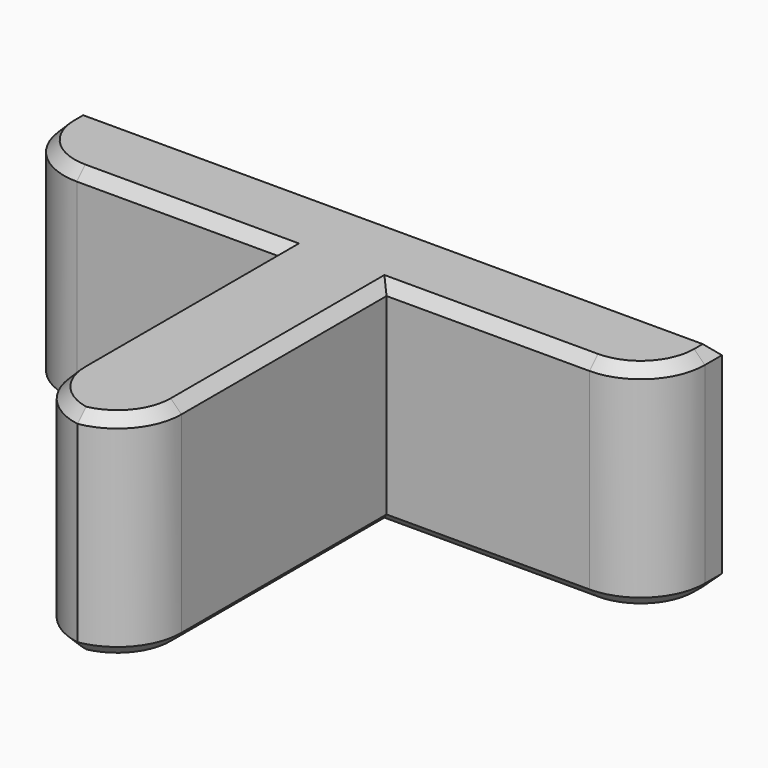
from build123d import *

# Parameters (mm, degrees)
F1_DEPTH    = 10
F2_T1_DEPTH = 25
F3_SIZE     = 0.5


# Not quite as in the source:
# - a fillet or chamfer that OpenCascade refuses, or shapes differently, is made with other operations: its cross-section is extruded or revolved along the edge and cut away or added


with BuildPart() as f1:
    # F0 (on Top) → F1 (new body)
    with BuildSketch(Plane.XY):
        Polygon((-15, 4), (-15, 0), (-2.5, 0), (-2.5, -15), (2.5, -15), (2.5, 0), (15, 0), (15, 4), align=None)
    extrude(amount=F1_DEPTH)

    # F2: fillet of radius 3 on 4 edges, made by hand

    # F2_s2 → F2_t1 (cut)
    with BuildSketch(Plane.XY.offset(-7.5)):
        with BuildLine():
            ThreePointArc((-2.5, -12), (-1.6213203436, -14.1213203436), (0.5, -15))
            Line((0.5, -15), (-2.5, -15))
            Line((-2.5, -15), (-2.5, -12))
        make_face()
        with BuildLine():
            ThreePointArc((-0.5, -15), (1.6213203436, -14.1213203436), (2.5, -12))
            Line((2.5, -12), (2.5, -15))
            Line((2.5, -15), (-0.5, -15))
        make_face()
        with BuildLine():
            ThreePointArc((-15, 3), (-14.1213203436, 0.8786796564), (-12, 0))
            Line((-12, 0), (-15, 0))
            Line((-15, 0), (-15, 3))
        make_face()
        with BuildLine():
            ThreePointArc((12, 0), (14.1213203436, 0.8786796564), (15, 3))
            Line((15, 3), (15, 0))
            Line((15, 0), (12, 0))
        make_face()
    extrude(amount=F2_T1_DEPTH, mode=Mode.SUBTRACT)

    # F3
    f3_edges = [f1.edges().sort_by_distance(p)[0] for p in [
        (0, 4, 10),
        (15, 3.5, 10),
        (14.12132, 0.87868, 10),
        (7.25, 0, 10),
        (2.5, -6, 10),
        (1.791288, -13.936492, 10),
        (-1.791288, -13.936492, 10),
        (-2.5, -6, 10),
        (-7.25, 0, 10),
        (-14.12132, 0.87868, 10),
        (-15, 3.5, 10),
        (0, 4, 0),
        (15, 3.5, 0),
        (14.12132, 0.87868, 0),
        (7.25, 0, 0),
        (2.5, -6, 0),
        (1.791288, -13.936492, 0),
        (-1.791288, -13.936492, 0),
        (-2.5, -6, 0),
        (-7.25, 0, 0),
        (-14.12132, 0.87868, 0),
        (-15, 3.5, 0),
    ]]
    chamfer(f3_edges, length=F3_SIZE)


solid = f1.part
